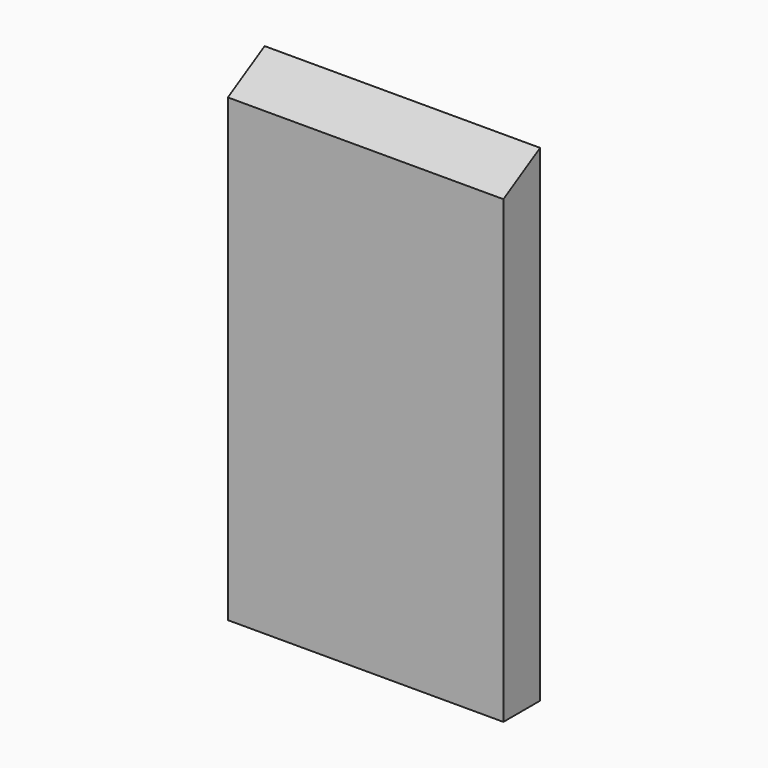
from build123d import *

# Parameters (mm, degrees)
F0_W     = 152.4
F0_H     = 269.24
F1_DEPTH = 25.4
F2_SIZE2 = 14.664687
F2_SIZE  = 25.39999


# Not quite as in the source:
# - a fillet or chamfer is up to 0.001 mm smaller than in the source, because OpenCascade refuses the exact size


with BuildPart() as f1:
    # F0 (on Front) → F1 (new body)
    with BuildSketch(Plane.XZ):
        with Locations((-1.5368815511, 8.3307931341)):
            Rectangle(F0_W, F0_H)
    extrude(amount=F1_DEPTH)

    # F2 (size 25.4 and 14.6646968374 in the source; OpenCascade refuses exactly that, so slightly less here)
    f2_edges = [f1.edges().sort_by_distance(p)[0] for p in [
        (-1.536882, -25.4, 142.950793),
    ]]
    f2_side = f1.faces().sort_by_distance((-1.536882, -12.7, 142.950793))[0]
    chamfer(f2_edges, length=F2_SIZE, length2=F2_SIZE2, reference=f2_side)


solid = f1.part
